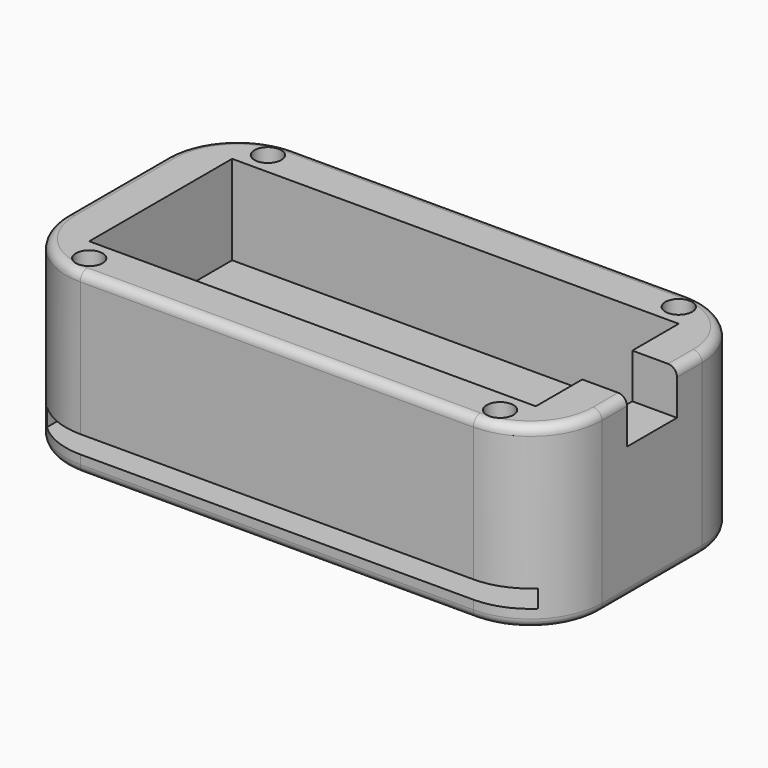
from build123d import *

# Parameters (mm, degrees)
F0_W          = 76.2
F0_H          = 38.1
F1_DEPTH      = 25.4
F2_W          = 69.85
F2_H          = 2.54
F3_DEPTH      = 38.101
F4_W          = 63.5
F4_H          = 25.4
F5_DEPTH      = 12.7
F6_W          = 6.35
F6_H          = 8.89
F7_DEPTH      = 6.35
F8_R          = 1.905
F9_DEPTH      = 6.35
F10_T1_DEPTH  = 76.2
F11_T1_DEPTH  = 17.78
F11_T3_DEPTH  = 55.88
F11_T5_DEPTH  = 7.62
F11_T7_DEPTH  = 7.62
F11_T10_ANGLE = 90.0000000017
F11_T12_ANGLE = 89.9999999998
F11_T14_ANGLE = 89.9999999979
F11_T16_ANGLE = 89.9999999998
F11_T18_ANGLE = 89.9999999998
F11_T20_ANGLE = 89.9999999998
F11_T22_ANGLE = 89.9999999979
F11_T24_ANGLE = 90.0000000017


# Not quite as in the source:
# - a fillet or chamfer that OpenCascade refuses, or shapes differently, is made with other operations: its cross-section is extruded or revolved along the edge and cut away or added


with BuildPart() as f1:
    # F0 (on Top) → F1 (new body)
    with BuildSketch(Plane.XY):
        with Locations((-11.0715073586, -8.5605031371)):
            Rectangle(F0_W, F0_H)
    extrude(amount=F1_DEPTH)

    # F2 (on face) → F3 (cut, through all)
    with BuildSketch(Plane.XZ.offset(27.6105031371)):
        with Locations((-11.0715073586, 3.81)):
            Rectangle(F2_W, F2_H)
    extrude(amount=-F3_DEPTH, mode=Mode.SUBTRACT)

    # F4 (on face) → F5 (cut)
    with BuildSketch(Plane.XY.offset(25.4)):
        with Locations((-11.0715073586, -8.5605031371)):
            Rectangle(F4_W, F4_H)
    extrude(amount=-F5_DEPTH, mode=Mode.SUBTRACT)

    # F6 (on face) → F7 (cut)
    with BuildSketch(Plane.XY.offset(25.4)):
        with Locations((23.8534926414, -8.5605031371)):
            Rectangle(F6_W, F6_H)
    extrude(amount=-F7_DEPTH, mode=Mode.SUBTRACT)

    # F8 (on face) → F9 (cut)
    with BuildSketch(Plane.XY.offset(25.4)):
        with Locations((-40.2815073586, 7.3144968629)):
            Circle(F8_R)
        with Locations((18.1384926414, 7.3144968629)):
            Circle(F8_R)
        with Locations((-40.2815073586, -24.4355031371)):
            Circle(F8_R)
        with Locations((18.1384926414, -24.4355031371)):
            Circle(F8_R)
    extrude(amount=-F9_DEPTH, mode=Mode.SUBTRACT)

    # F10: fillet of radius 10.16 on 4 edges, made by hand

    # F10_s2 → F10_t1 (cut)
    with BuildSketch(Plane.XY.offset(-25.4)):
        with BuildLine():
            ThreePointArc((-39.0115073586, -27.6105031371), (-46.1957122554, -24.634708034), (-49.1715073586, -17.4505031371))
            Line((-49.1715073586, -17.4505031371), (-49.1715073586, -27.6105031371))
            Line((-49.1715073586, -27.6105031371), (-39.0115073586, -27.6105031371))
        make_face()
        with BuildLine():
            ThreePointArc((27.0284926414, -17.4505031371), (24.0526975383, -24.634708034), (16.8684926414, -27.6105031371))
            Line((16.8684926414, -27.6105031371), (27.0284926414, -27.6105031371))
            Line((27.0284926414, -27.6105031371), (27.0284926414, -17.4505031371))
        make_face()
        with BuildLine():
            ThreePointArc((27.0284926414, 0.3294968629), (24.0526975383, 7.5137017597), (16.8684926414, 10.4894968629))
            Line((16.8684926414, 10.4894968629), (27.0284926414, 10.4894968629))
            Line((27.0284926414, 10.4894968629), (27.0284926414, 0.3294968629))
        make_face()
        with BuildLine():
            ThreePointArc((-39.0115073586, 10.4894968629), (-46.1957122554, 7.5137017597), (-49.1715073586, 0.3294968629))
            Line((-49.1715073586, 0.3294968629), (-49.1715073586, 10.4894968629))
            Line((-49.1715073586, 10.4894968629), (-39.0115073586, 10.4894968629))
        make_face()
    extrude(amount=F10_T1_DEPTH, mode=Mode.SUBTRACT)

    # F11: fillet of radius 1.27 on 17 edges, made by hand

    # F11_s2 → F11_t1 (cut)
    with BuildSketch(Plane.XZ.offset(-0.3294968629)):
        with BuildLine():
            ThreePointArc((-47.9015073586, 25.4), (-48.7995329707, 25.0280256121), (-49.1715073586, 24.13))
            Line((-49.1715073586, 24.13), (-49.1715073586, 25.4))
            Line((-49.1715073586, 25.4), (-47.9015073586, 25.4))
        make_face()
        with BuildLine():
            ThreePointArc((27.0284926414, 1.27), (26.6565182536, 0.3719743879), (25.7584926414, 0))
            Line((25.7584926414, 0), (27.0284926414, 0))
            Line((27.0284926414, 0), (27.0284926414, 1.27))
        make_face()
        with BuildLine():
            ThreePointArc((-47.9015073586, 0), (-48.7995329707, 0.3719743879), (-49.1715073586, 1.27))
            Line((-49.1715073586, 1.27), (-49.1715073586, 0))
            Line((-49.1715073586, 0), (-47.9015073586, 0))
        make_face()
    extrude(amount=F11_T1_DEPTH, mode=Mode.SUBTRACT)

    # F11_s4 → F11_t3 (cut)
    with BuildSketch(Plane.YZ.offset(-39.0115073586)):
        with BuildLine():
            ThreePointArc((9.2194968629, 0), (10.117522475, 0.3719743879), (10.4894968629, 1.27))
            Line((10.4894968629, 1.27), (10.4894968629, 0))
            Line((10.4894968629, 0), (9.2194968629, 0))
        make_face()
        with BuildLine():
            ThreePointArc((-26.3405031371, 0), (-27.2385287492, 0.3719743879), (-27.6105031371, 1.27))
            Line((-27.6105031371, 1.27), (-27.6105031371, 0))
            Line((-27.6105031371, 0), (-26.3405031371, 0))
        make_face()
        with BuildLine():
            ThreePointArc((9.2194968629, 25.4), (10.117522475, 25.0280256121), (10.4894968629, 24.13))
            Line((10.4894968629, 24.13), (10.4894968629, 25.4))
            Line((10.4894968629, 25.4), (9.2194968629, 25.4))
        make_face()
        with BuildLine():
            ThreePointArc((-26.3405031371, 25.4), (-27.2385287492, 25.0280256121), (-27.6105031371, 24.13))
            Line((-27.6105031371, 24.13), (-27.6105031371, 25.4))
            Line((-27.6105031371, 25.4), (-26.3405031371, 25.4))
        make_face()
    extrude(amount=F11_T3_DEPTH, mode=Mode.SUBTRACT)

    # F11_s6 → F11_t5 (cut)
    with BuildSketch(Plane.XZ.offset(-0.3294968629)):
        with BuildLine():
            ThreePointArc((27.0284926414, 24.13), (26.6565182536, 25.0280256121), (25.7584926414, 25.4))
            Line((25.7584926414, 25.4), (27.0284926414, 25.4))
            Line((27.0284926414, 25.4), (27.0284926414, 24.13))
        make_face()
    extrude(amount=F11_T5_DEPTH, mode=Mode.SUBTRACT)

    # F11_s8 → F11_t7 (cut)
    with BuildSketch(Plane.XZ.offset(9.8305031371)):
        with BuildLine():
            ThreePointArc((27.0284926414, 24.13), (26.6565182536, 25.0280256121), (25.7584926414, 25.4))
            Line((25.7584926414, 25.4), (27.0284926414, 25.4))
            Line((27.0284926414, 25.4), (27.0284926414, 24.13))
        make_face()
    extrude(amount=F11_T7_DEPTH, mode=Mode.SUBTRACT)

    # F11_s9 → F11_t10 (revolve, cut)
    with BuildSketch(Plane.XZ.offset(17.4505031373)):
        with BuildLine():
            ThreePointArc((25.7584926414, 0), (26.6565182535, 0.3719743879), (27.0284926414, 1.27))
            Line((27.0284926414, 1.27), (27.0284926414, 0))
            Line((27.0284926414, 0), (25.7584926414, 0))
        make_face()
    revolve(axis=Axis((16.8684926416, -17.4505031373, 0), (0, 0, -1)), revolution_arc=F11_T10_ANGLE, mode=Mode.SUBTRACT)

    # F11_s11 → F11_t12 (revolve, cut)
    with BuildSketch(Plane.YZ.offset(-39.0115073586)):
        with BuildLine():
            ThreePointArc((-26.3405031371, 0), (-27.2385287492, 0.3719743879), (-27.6105031371, 1.27))
            Line((-27.6105031371, 1.27), (-27.6105031371, 0))
            Line((-27.6105031371, 0), (-26.3405031371, 0))
        make_face()
    revolve(axis=Axis((-39.0115073586, -17.4505031371, 0), (0, 0, -1)), revolution_arc=F11_T12_ANGLE, mode=Mode.SUBTRACT)

    # F11_s13 → F11_t14 (revolve, cut)
    with BuildSketch(Plane.XZ.offset(-0.3294968627)):
        with BuildLine():
            ThreePointArc((-47.9015073586, 0), (-48.7995329707, 0.3719743879), (-49.1715073586, 1.27))
            Line((-49.1715073586, 1.27), (-49.1715073586, 0))
            Line((-49.1715073586, 0), (-47.9015073586, 0))
        make_face()
    revolve(axis=Axis((-39.0115073584, 0.3294968627, 0), (0, 0, -1)), revolution_arc=F11_T14_ANGLE, mode=Mode.SUBTRACT)

    # F11_s15 → F11_t16 (revolve, cut)
    with BuildSketch(Plane.YZ.offset(16.8684926414)):
        with BuildLine():
            ThreePointArc((9.2194968629, 0), (10.117522475, 0.3719743879), (10.4894968629, 1.27))
            Line((10.4894968629, 1.27), (10.4894968629, 0))
            Line((10.4894968629, 0), (9.2194968629, 0))
        make_face()
    revolve(axis=Axis((16.8684926414, 0.3294968629, 0), (0, 0, -1)), revolution_arc=F11_T16_ANGLE, mode=Mode.SUBTRACT)

    # F11_s17 → F11_t18 (revolve, cut)
    with BuildSketch(Plane.YZ.offset(16.8684926414)):
        with BuildLine():
            ThreePointArc((10.4894968629, 24.13), (10.117522475, 25.0280256121), (9.2194968629, 25.4))
            Line((9.2194968629, 25.4), (10.4894968629, 25.4))
            Line((10.4894968629, 25.4), (10.4894968629, 24.13))
        make_face()
    revolve(axis=Axis((16.8684926414, 0.3294968629, 25.4), (0, 0, -1)), revolution_arc=F11_T18_ANGLE, mode=Mode.SUBTRACT)

    # F11_s19 → F11_t20 (revolve, cut)
    with BuildSketch(Plane.YZ.offset(-39.0115073586)):
        with BuildLine():
            ThreePointArc((-26.3405031371, 25.4), (-27.2385287492, 25.0280256121), (-27.6105031371, 24.13))
            Line((-27.6105031371, 24.13), (-27.6105031371, 25.4))
            Line((-27.6105031371, 25.4), (-26.3405031371, 25.4))
        make_face()
    revolve(axis=Axis((-39.0115073586, -17.4505031371, 25.4), (0, 0, -1)), revolution_arc=F11_T20_ANGLE, mode=Mode.SUBTRACT)

    # F11_s21 → F11_t22 (revolve, cut)
    with BuildSketch(Plane.XZ.offset(-0.3294968627)):
        with BuildLine():
            ThreePointArc((-47.9015073586, 25.4), (-48.7995329707, 25.0280256121), (-49.1715073586, 24.13))
            Line((-49.1715073586, 24.13), (-49.1715073586, 25.4))
            Line((-49.1715073586, 25.4), (-47.9015073586, 25.4))
        make_face()
    revolve(axis=Axis((-39.0115073584, 0.3294968627, 25.4), (0, 0, -1)), revolution_arc=F11_T22_ANGLE, mode=Mode.SUBTRACT)

    # F11_s23 → F11_t24 (revolve, cut)
    with BuildSketch(Plane.XZ.offset(17.4505031373)):
        with BuildLine():
            ThreePointArc((25.7584926414, 25.4), (26.6565182535, 25.0280256121), (27.0284926414, 24.13))
            Line((27.0284926414, 24.13), (27.0284926414, 25.4))
            Line((27.0284926414, 25.4), (25.7584926414, 25.4))
        make_face()
    revolve(axis=Axis((16.8684926416, -17.4505031373, 25.4), (0, 0, -1)), revolution_arc=F11_T24_ANGLE, mode=Mode.SUBTRACT)


solid = f1.part
